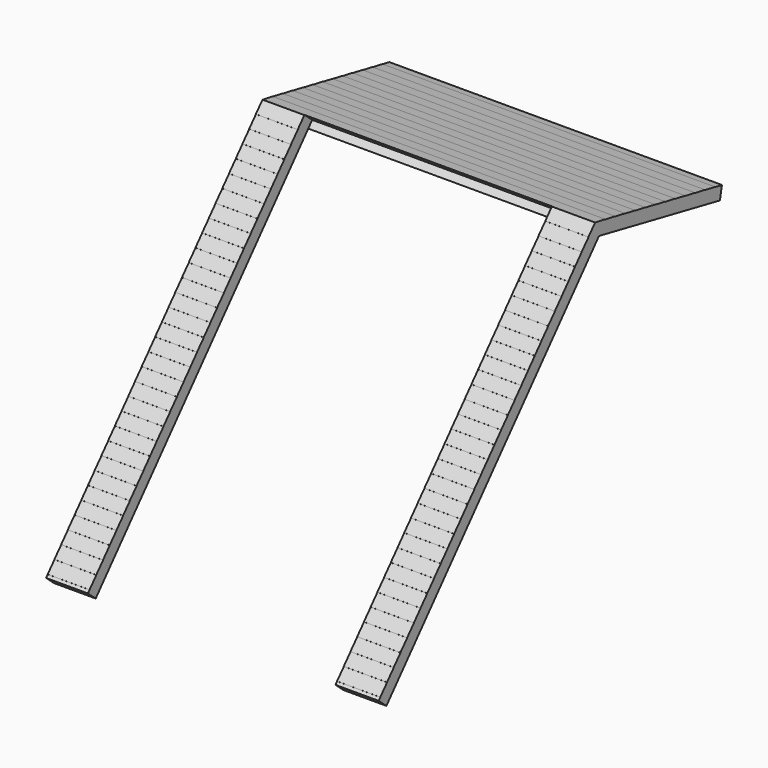
from build123d import *

# Parameters (mm, degrees)
F1_DEPTH = 3962.4
F2_W     = 982.98
F2_H     = 4914.9
F3_DEPTH = 154.178
F5_DEPTH = 3962.4


# Not quite as in the source:
# - ends of sketch curves that miss each other by under 0.0002 mm in the source are joined


with BuildPart() as f1:
    # F0 (on Right) → F1 (new body)
    with BuildSketch(Plane.YZ):
        Polygon((-1062.7204243511, -1222.520001882), (0, 0), (1800.8836783461, -359.1330239131), (1831.0362082596, -207.9322282015), (-57.6330628745, 168.7070376599), (-3282.0975844599, -3540.615078177), (-3165.7379708004, -3641.7649471487), align=None)
    extrude(amount=F1_DEPTH)

    # F2 (on face) → F3 (cut)
    with BuildSketch(Plane(origin=(0, -116.3596136596, 101.1498689717), x_dir=(1, 0, 0), z_dir=(0, -0.7547095802, 0.656059029))):
        Polygon((1481.7409789185, -4825.3858736942), (1481.7409789185, 89.5141263058), (498.7609789185, 89.5141263058), (498.7609789185, -1548.7858736942), (498.7609789185, -3187.0858736942), (498.7609789185, -4825.3858736942), align=None)
        with Locations((1973.2309789185, -2367.9358736942)):
            Rectangle(F2_W, F2_H)
        with Locations((2956.2109789185, -2367.9358736942)):
            Rectangle(F2_W, F2_H)
    extrude(amount=-F3_DEPTH, mode=Mode.SUBTRACT)

    # F4 (on face) → F5 (cut)
    with BuildSketch(Plane(origin=(0, 0, 0), x_dir=(0, -1, 0), z_dir=(-1, 0, 0))):
        Polygon((3359.7929958838, -3626.122896465), (3257.9070493635, -3512.7870508483), (3256.0181183313, -3514.4851502014), align=None)
        Polygon((-1728.0633988919, -189.9869954259), (-1728.5183752228, -187.4880763519), (-1877.975504427, -217.2928835151), align=None)
        Polygon((157.6164588926, 53.689297634), (57.6330628745, 168.7070376599), (57.6330628745, 164.9077501103), align=None)
        Polygon((57.6330628745, 164.9077501103), (57.6330628745, 168.7070376599), (-91.8240663297, 138.9022304967), align=None)
        Polygon((257.5998549108, -61.328442392), (157.6164588926, 53.689297634), (155.6994965589, 52.0229077003), align=None)
        Polygon((357.5832509291, -176.3461824181), (257.5998549108, -61.328442392), (255.682892577, -62.9948323256), align=None)
        Polygon((457.5944201085, -291.3958718113), (357.5832509291, -176.3461824181), (355.6943240939, -178.0442858929), align=None)
        Polygon((557.6055854343, -406.4455567714), (457.5944201085, -291.3958718113), (455.7054893441, -293.0939709155), align=None)
        Polygon((657.6167507599, -521.4952417314), (557.6055854343, -406.4455567714), (555.7166546943, -408.1436558504), align=None)
        Polygon((757.6279160871, -636.5449266932), (657.6167507599, -521.4952417314), (655.7278198727, -523.1933409397), align=None)
        Polygon((857.6390814104, -751.5946116505), (757.6279160871, -636.5449266932), (755.7389850512, -638.2430260291), align=None)
        Polygon((957.6502467357, -866.64429661), (857.6390814104, -751.5946116505), (855.7501502296, -753.2927111184), align=None)
        Polygon((1057.6614120711, -981.6939815812), (957.6502467357, -866.64429661), (955.7613154081, -868.3423962077), align=None)
        Polygon((1157.6725773853, -1096.743666528), (1057.6614120711, -981.6939815812), (1055.7724803196, -983.3920815471), align=None)
        Polygon((1257.6837427263, -1211.7933515057), (1157.6725773853, -1096.743666528), (1155.7836463636, -1098.4417658929), align=None)
        Polygon((1357.694908057, -1326.8430364714), (1257.6837427263, -1211.7933515057), (1255.7948116941, -1213.4914508588), align=None)
        Polygon((1457.7060733877, -1441.8927214372), (1357.694908057, -1326.8430364714), (1355.8059770247, -1328.5411358246), align=None)
        Polygon((1557.7172387183, -1556.942406403), (1457.7060733877, -1441.8927214372), (1455.8171423554, -1443.5908207904), align=None)
        Polygon((1657.728404049, -1671.9920913688), (1557.7172387183, -1556.942406403), (1555.8283076861, -1558.6405057562), align=None)
        Polygon((1957.7619000458, -2017.1411462715), (1857.7507347135, -1902.0914613039), (1855.8618036813, -1903.7895606571), align=None)
        Polygon((1857.7507347135, -1902.0914613039), (1757.7395693813, -1787.0417763363), (1755.850638349, -1788.7398756895), align=None)
        Polygon((1757.7395693813, -1787.0417763363), (1657.728404049, -1671.9920913688), (1655.8394730168, -1673.6901907219), align=None)
        Polygon((2057.773065378, -2132.1908312391), (1957.7619000458, -2017.1411462715), (1955.8729690135, -2018.8392456247), align=None)
        Polygon((2157.7842307103, -2247.2405162067), (2057.773065378, -2132.1908312391), (2055.8841343458, -2133.8889305922), align=None)
        Polygon((2257.7953960425, -2362.2902011743), (2157.7842307103, -2247.2405162067), (2155.895299678, -2248.9386155598), align=None)
        Polygon((2357.8065613748, -2477.3398861418), (2257.7953960425, -2362.2902011743), (2255.9064650103, -2363.9883005274), align=None)
        Polygon((2457.817726707, -2592.3895711094), (2357.8065613748, -2477.3398861418), (2355.9176303426, -2479.037985495), align=None)
        Polygon((2557.8288920393, -2707.439256077), (2457.817726707, -2592.3895711094), (2455.9287956748, -2594.0876704626), align=None)
        Polygon((2657.8400573716, -2822.4889410446), (2557.8288920393, -2707.439256077), (2555.9399610071, -2709.1373554302), align=None)
        Polygon((2655.9511263393, -2824.1870403977), (2757.8512227038, -2937.5386260122), (2657.8400573716, -2822.4889410446), align=None)
        Polygon((2755.9622916716, -2939.2367253653), (2857.8623880361, -3052.5883109797), (2757.8512227038, -2937.5386260122), align=None)
        Polygon((2855.9734570038, -3054.2864103329), (2957.8735533683, -3167.6379959473), (2857.8623880361, -3052.5883109797), align=None)
        Polygon((2955.9846223361, -3169.3360953005), (3057.8847187006, -3282.6876809149), (2957.8735533683, -3167.6379959473), align=None)
        Polygon((3055.9957876683, -3284.3857802681), (3157.8958840328, -3397.7373658825), (3057.8847187006, -3282.6876809149), align=None)
        Polygon((3156.0069530006, -3399.4354652356), (3257.9070493635, -3512.7870508483), (3157.8958840328, -3397.7373658825), align=None)
        Polygon((-1579.2692161887, -160.3143933487), (-1579.7241925196, -157.8154742747), (-1728.5183752228, -187.4880763519), align=None)
        Polygon((-1430.4750334855, -130.6417912715), (-1430.9300098164, -128.1428721975), (-1579.7241925196, -157.8154742747), align=None)
        Polygon((-1281.6808507823, -100.9691891943), (-1282.1358271132, -98.4702701204), (-1430.9300098164, -128.1428721975), align=None)
        Polygon((-1132.8866680792, -71.2965871171), (-1133.34164441, -68.7976680432), (-1282.1358271132, -98.4702701204), align=None)
        Polygon((-984.092485376, -41.62398504), (-984.5474617069, -39.125065966), (-1133.34164441, -68.7976680432), align=None)
        Polygon((-835.2983026728, -11.9513829628), (-835.7532790037, -9.4524638888), (-984.5474617069, -39.125065966), align=None)
        Polygon((-686.5041199696, 17.7212191144), (-686.9590963005, 20.2201381884), (-835.7532790037, -9.4524638888), align=None)
        Polygon((-537.7099372664, 47.3938211916), (-538.1649135973, 49.8927402656), (-686.9590963005, 20.2201381884), align=None)
        Polygon((-388.9157545632, 77.0664232688), (-389.3707308958, 79.5653423425), (-538.1649135973, 49.8927402656), align=None)
        Polygon((-240.1215718796, 106.7390254439), (-240.5765423462, 109.2379455855), (-389.3707308958, 79.5653423425), align=None)
        Polygon((-91.3273195437, 136.4112783433), (-91.8240663297, 138.9022304967), (-240.5765423462, 109.2379455855), align=None)
    extrude(amount=-F5_DEPTH, mode=Mode.SUBTRACT)


solid = f1.part
